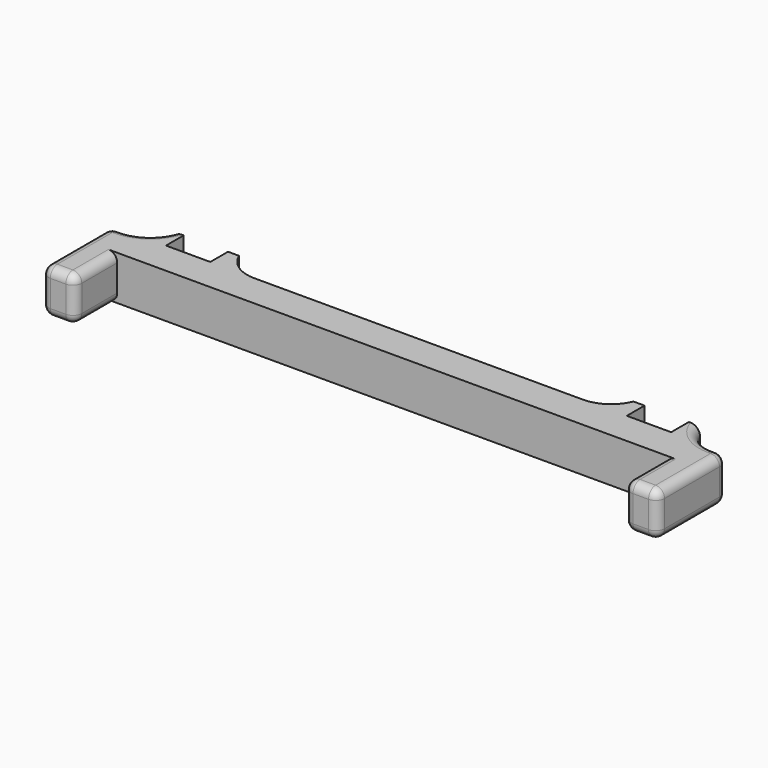
from build123d import *

# Parameters (mm, degrees)
F1_DEPTH    = 6.35
F2_T1_DEPTH = 6.35
F3_R        = 1.27


# Not quite as in the source:
# - a fillet or chamfer that OpenCascade refuses, or shapes differently, is made with other operations: its cross-section is extruded or revolved along the edge and cut away or added


with BuildPart() as f1:
    # F0 (on Top) → F1 (new body)
    with BuildSketch(Plane.XY):
        Polygon((28.2575, 0), (0, 0), (0, -4.7625), (39.37, -4.7625), (39.37, -12.3825), (44.1325, -12.3825), (44.1325, 0), (37.7825, 0), (37.7825, 3.175), (36.195, 3.175), (36.195, 0), (29.845, 0), (29.845, 3.175), (28.2575, 3.175), align=None)
    extrude(amount=F1_DEPTH)

    # F2: fillet of radius 5.08 on 2 edges, made by hand

    # F2_s2 → F2_t1 (join)
    with BuildSketch(Plane.XY):
        with BuildLine():
            ThreePointArc((42.4917860393, 0), (39.6519797079, 0.8678865162), (37.7825, 3.175))
            Line((37.7825, 3.175), (37.7825, 0))
            Line((37.7825, 0), (42.4917860393, 0))
        make_face()
        with BuildLine():
            ThreePointArc((23.5482139607, 0), (26.3880202921, 0.8678865162), (28.2575, 3.175))
            Line((28.2575, 3.175), (28.2575, 0))
            Line((28.2575, 0), (23.5482139607, 0))
        make_face()
    extrude(amount=F2_T1_DEPTH)

    # F3
    f3_edges = [f1.edges().sort_by_distance(p)[0] for p in [
        (39.37, -8.5725, 0),
        (44.1325, -6.19125, 6.35),
        (41.75125, -12.3825, 6.35),
        (44.1325, -12.3825, 3.175),
        (39.37, -12.3825, 3.175),
        (41.75125, -12.3825, 0),
        (39.37, -8.5725, 6.35),
        (44.1325, -6.19125, 0),
        (39.65198, 0.867887, 6.35),
        (39.65198, 0.867887, 0),
        (43.312143, 0, 6.35),
        (43.312143, 0, 0),
        (44.1325, 0, 3.175),
    ]]
    fillet(f3_edges, radius=F3_R)

    # F4: F1 across plane


with BuildPart() as f1_1:
    add(f1.part)
    add(f1.part.mirror(Plane.YZ))


solid = f1_1.part
